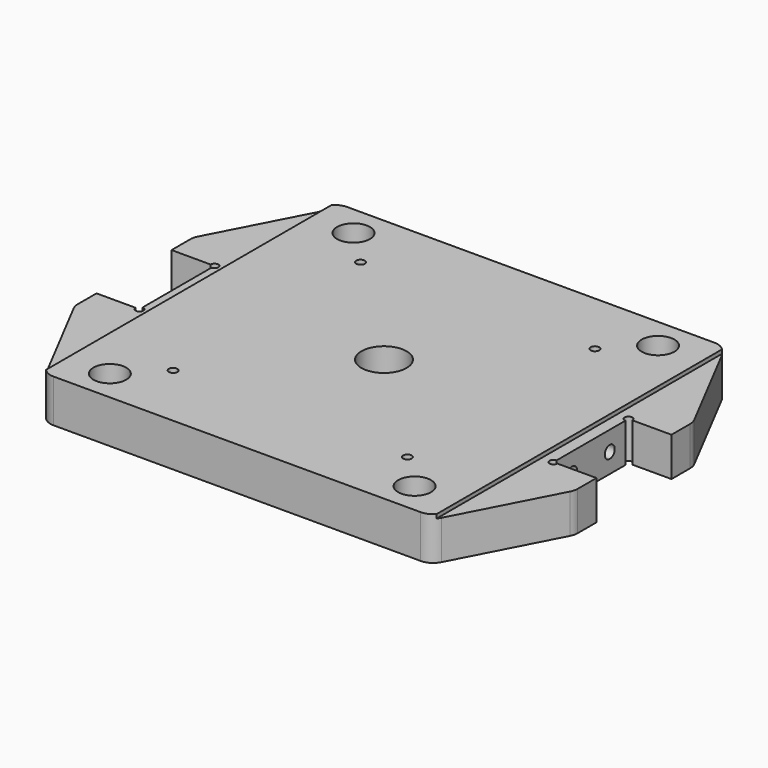
from build123d import *

# Parameters (mm, degrees)
F0_R     = 35
F0_R_2   = 5.5
F0_R_3   = 50
F0_R_4   = 29
F0_R_5   = 21
F1_DEPTH = 55
F2_DEPTH = 10
F4_DEPTH = 5
F5_R     = 8
F6_DEPTH = 25
F7_R     = 8
F8_DEPTH = 25


# Not quite as in the source:
# - ends of sketch curves that miss each other by under 0.0002 mm in the source are joined


with BuildPart() as f1:
    # F0 (on Top) → F1 (new body)
    with BuildSketch(Plane.XY):
        with BuildLine():
            ThreePointArc((-265, -55), (-261.4644660941, -63.5355339059), (-270, -60))
            Line((-270, -60), (-320, -60))
            Line((-320, -60), (-320, -90))
            ThreePointArc((-320, -90), (-319.427901562, -94.7493832125), (-317.7443359101, -99.2270549532))
            Line((-317.7443359101, -99.2270549532), (-252.744336, -224.227055))
            ThreePointArc((-252.744336, -224.227055), (-245.3792798627, -232.0959220147), (-235, -235))
            Line((-235, -235), (235, -235))
            ThreePointArc((235, -235), (245.3792798627, -232.0959220147), (252.7443359101, -224.2270549532))
            Line((252.7443359101, -224.2270549532), (317.744336, -99.227055))
            ThreePointArc((317.744336, -99.227055), (319.427901562, -94.7493832125), (320, -90))
            Line((320, -90), (320, -60))
            Line((320, -60), (270, -60))
            ThreePointArc((270, -60), (261.4644660941, -63.5355339059), (265, -55))
            Line((265, -55), (265, 55))
            ThreePointArc((265, 55), (261.4644660941, 63.5355339059), (270, 60))
            Line((270, 60), (320, 60))
            Line((320, 60), (320, 90))
            ThreePointArc((320, 90), (319.427901562, 94.7493832125), (317.7443359101, 99.2270549532))
            Line((317.7443359101, 99.2270549532), (252.744336, 224.227055))
            ThreePointArc((252.744336, 224.227055), (245.3792798627, 232.0959220147), (235, 235))
            Line((235, 235), (-235, 235))
            ThreePointArc((-235, 235), (-245.3792798627, 232.0959220147), (-252.7443359101, 224.2270549532))
            Line((-252.7443359101, 224.2270549532), (-317.744336, 99.227055))
            ThreePointArc((-317.744336, 99.227055), (-319.427901562, 94.7493832125), (-320, 90))
            Line((-320, 90), (-320, 60))
            Line((-320, 60), (-270, 60))
            ThreePointArc((-270, 60), (-261.4644660941, 63.5355339059), (-265, 55))
            Line((-265, 55), (-265, -55))
        make_face()
        with Locations((-195, -195)):
            Circle(F0_R, mode=Mode.SUBTRACT)
        with Locations((-150, -150)):
            Circle(F0_R_2, mode=Mode.SUBTRACT)
        with Locations((150, -150)):
            Circle(F0_R_2, mode=Mode.SUBTRACT)
        with Locations((195, -194.81006)):
            Circle(F0_R, mode=Mode.SUBTRACT)
        with Locations((0, -0.1899)):
            Circle(F0_R_3, mode=Mode.SUBTRACT)
        with Locations((-195, 195)):
            Circle(F0_R, mode=Mode.SUBTRACT)
        with Locations((-150, 150)):
            Circle(F0_R_2, mode=Mode.SUBTRACT)
        with Locations((150, 150)):
            Circle(F0_R_2, mode=Mode.SUBTRACT)
        with Locations((195, 194.810059)):
            Circle(F0_R, mode=Mode.SUBTRACT)
        with Locations((0, -0.1899)):
            Circle(F0_R_3)
        with Locations((0, 4e-05)):
            Circle(F0_R_4, mode=Mode.SUBTRACT)
        with Locations((-195, 195)):
            Circle(F0_R)
        with Locations((-195, 195)):
            Circle(F0_R_5, mode=Mode.SUBTRACT)
        with Locations((195, 194.810059)):
            Circle(F0_R)
        with Locations((195, 194.810059)):
            Circle(F0_R_5, mode=Mode.SUBTRACT)
        with Locations((-195, -195)):
            Circle(F0_R)
        with Locations((-195, -195)):
            Circle(F0_R_5, mode=Mode.SUBTRACT)
        with Locations((195, -194.81006)):
            Circle(F0_R)
        with Locations((195, -194.81006)):
            Circle(F0_R_5, mode=Mode.SUBTRACT)
    extrude(amount=F1_DEPTH)

    # F0 (on Top) → F2 (cut)
    with BuildSketch(Plane.XY):
        with Locations((195, 194.810059)):
            Circle(F0_R)
        with Locations((195, 194.810059)):
            Circle(F0_R_5, mode=Mode.SUBTRACT)
        with Locations((-195, 195)):
            Circle(F0_R)
        with Locations((-195, 195)):
            Circle(F0_R_5, mode=Mode.SUBTRACT)
        with Locations((0, -0.1899)):
            Circle(F0_R_3)
        with Locations((0, 4e-05)):
            Circle(F0_R_4, mode=Mode.SUBTRACT)
        with Locations((-195, -195)):
            Circle(F0_R)
        with Locations((-195, -195)):
            Circle(F0_R_5, mode=Mode.SUBTRACT)
        with Locations((195, -194.81006)):
            Circle(F0_R)
        with Locations((195, -194.81006)):
            Circle(F0_R_5, mode=Mode.SUBTRACT)
    extrude(amount=F2_DEPTH, mode=Mode.SUBTRACT)

    # F3 (on face) → F4 (cut)
    with BuildSketch(Plane.XY.offset(55)):
        with BuildLine():
            Line((270, 60), (320, 60))
            Line((320, 60), (320, 90))
            ThreePointArc((320, 90), (319.427901562, 94.7493832125), (317.7443359101, 99.2270549532))
            Line((317.7443359101, 99.2270549532), (252.744336, 224.227055))
            ThreePointArc((252.744336, 224.227055), (251.4939773544, 226.311441724), (250, 228.2287566232))
            Line((250, 228.2287566232), (250, -228.2287565553))
            ThreePointArc((250, -228.2287565553), (251.4939773092, -226.3114416643), (252.7443359101, -224.2270549532))
            Line((252.7443359101, -224.2270549532), (317.744336, -99.227055))
            ThreePointArc((317.744336, -99.227055), (319.4279015605, -94.7493832184), (320, -90))
            Line((320, -90), (320, -60))
            Line((320, -60), (270, -60))
            ThreePointArc((270, -60), (261.4644660941, -63.5355339059), (265, -55))
            Line((265, -55), (265, 55))
            ThreePointArc((265, 55), (261.4644660941, 63.5355339059), (270, 60))
        make_face()
        with BuildLine():
            Line((-250, -228.2287566232), (-250, 228.2287565553))
            ThreePointArc((-250, 228.2287565553), (-251.4939773092, 226.3114416643), (-252.7443359101, 224.2270549532))
            Line((-252.7443359101, 224.2270549532), (-317.744336, 99.227055))
            ThreePointArc((-317.744336, 99.227055), (-319.4279015605, 94.7493832184), (-320, 90))
            Line((-320, 90), (-320, 60))
            Line((-320, 60), (-270, 60))
            ThreePointArc((-270, 60), (-261.4644660941, 63.5355339059), (-265, 55))
            Line((-265, 55), (-265, -55))
            ThreePointArc((-265, -55), (-261.4644660941, -63.5355339059), (-270, -60))
            Line((-270, -60), (-320, -60))
            Line((-320, -60), (-320, -90))
            ThreePointArc((-320, -90), (-319.427901562, -94.7493832125), (-317.7443359101, -99.2270549532))
            Line((-317.7443359101, -99.2270549532), (-252.744336, -224.227055))
            ThreePointArc((-252.744336, -224.227055), (-251.4939773544, -226.311441724), (-250, -228.2287566232))
        make_face()
    extrude(amount=-F4_DEPTH, mode=Mode.SUBTRACT)

    # F5 (on face) → F6 (cut)
    with BuildSketch(Plane.YZ.offset(265)):
        with Locations((30, 25)):
            Circle(F5_R)
        with Locations((-30, 25)):
            Circle(F5_R)
    extrude(amount=-F6_DEPTH, mode=Mode.SUBTRACT)

    # F7 (on face) → F8 (cut)
    with BuildSketch(Plane(origin=(-265, 0, 0), x_dir=(0, -1, 0), z_dir=(-1, 0, 0))):
        with Locations((-30, 25)):
            Circle(F7_R)
        with Locations((30, 25)):
            Circle(F7_R)
    extrude(amount=-F8_DEPTH, mode=Mode.SUBTRACT)


solid = f1.part
